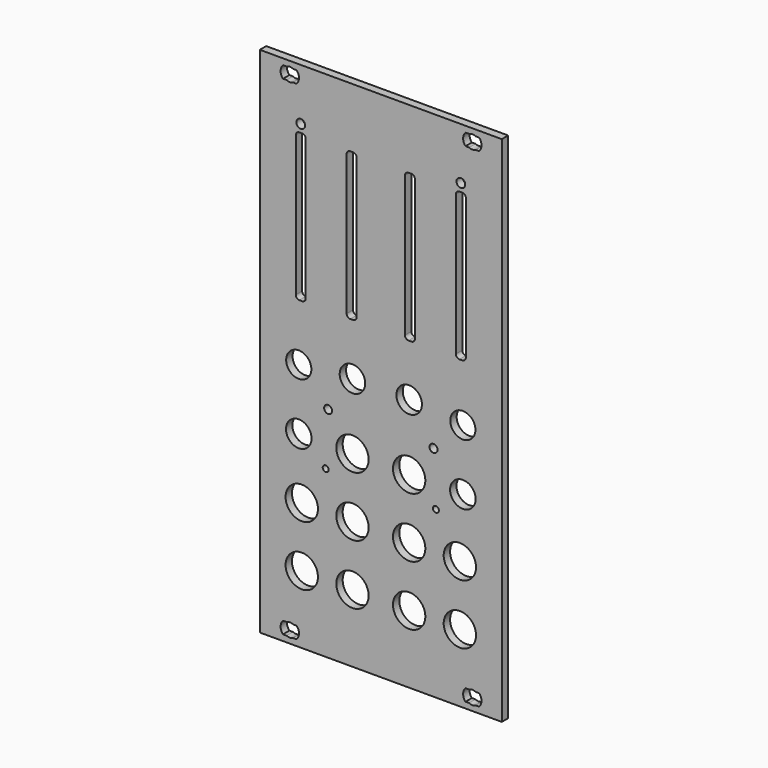
from build123d import *

# Parameters (mm, degrees)
F0_R     = 4.05
F0_R_2   = 3.200001
F0_R_3   = 3.15
F0_R_4   = 0.75
F0_R_5   = 1
F0_R_6   = 1.1
F1_DEPTH = 2


# Not quite as in the source:
# - ends of sketch curves that miss each other by under 0.0002 mm in the source are joined


with BuildPart() as f1:
    # F0 (on Front) → F1 (new body)
    with BuildSketch(Plane.XZ):
        Polygon((-30.3, -61.250013), (-30.3, -64.250012), (30.300001, -64.250012), (30.300001, 64.250011), (-30.3, 64.250011), align=None)
        with BuildLine():
            ThreePointArc((-23.600001, -59.750013), (-22.7999995588, -59.550011), (-21.9999982215, -59.7500134152))
            Line((-21.9999982215, -59.7500134152), (-21.100001, -59.750013))
            ThreePointArc((-21.100001, -59.750013), (-20.5, -61.2500126379), (-21.1000001998, -62.7500108097))
            Line((-21.1000001998, -62.7500108097), (-21.999999, -62.750012))
            ThreePointArc((-21.999999, -62.750012), (-22.7999995588, -62.950014), (-23.600001, -62.750012))
            Line((-23.600001, -62.750012), (-24.499999, -62.750012))
            ThreePointArc((-24.499999, -62.750012), (-25.1, -61.2500126379), (-24.4999988252, -59.7500141665))
            Line((-24.4999988252, -59.7500141665), (-23.600001, -59.750013))
        make_face(mode=Mode.SUBTRACT)
        with Locations((-19.800001, -47.249931)):
            Circle(F0_R, mode=Mode.SUBTRACT)
        with Locations((-19.800052, -32.249984)):
            Circle(F0_R, mode=Mode.SUBTRACT)
        with Locations((-7.100001, -47.249931)):
            Circle(F0_R, mode=Mode.SUBTRACT)
        with Locations((-7.100052, -32.249984)):
            Circle(F0_R, mode=Mode.SUBTRACT)
        with Locations((-20.549999, -17.249989)):
            Circle(F0_R_2, mode=Mode.SUBTRACT)
        with Locations((-20.549999, -1.999989)):
            Circle(F0_R_3, mode=Mode.SUBTRACT)
        with Locations((-13.8, -22.749991)):
            Circle(F0_R_4, mode=Mode.SUBTRACT)
        with Locations((-7.100052, -17.249986)):
            Circle(F0_R, mode=Mode.SUBTRACT)
        with Locations((-13.200001, -9.499989)):
            Circle(F0_R_5, mode=Mode.SUBTRACT)
        with Locations((-7.100001, -0.749989)):
            Circle(F0_R_2, mode=Mode.SUBTRACT)
        with Locations((7.099976, -47.249957)):
            Circle(F0_R, mode=Mode.SUBTRACT)
        with Locations((7.09995, -32.249928)):
            Circle(F0_R, mode=Mode.SUBTRACT)
        with BuildLine():
            ThreePointArc((22.119986, -59.750023), (22.9199874412, -59.550021), (23.7199887785, -59.7500234152))
            Line((23.7199887785, -59.7500234152), (24.619987, -59.750023))
            ThreePointArc((24.619987, -59.750023), (25.219987, -61.250023), (24.6199863008, -62.7500213341))
            Line((24.6199863008, -62.7500213341), (23.719988, -62.750022))
            ThreePointArc((23.719988, -62.750022), (22.9199874412, -62.950024), (22.119986, -62.750022))
            Line((22.119986, -62.750022), (21.219988, -62.750022))
            ThreePointArc((21.219988, -62.750022), (20.619987, -61.250023), (21.2199901249, -59.7500221189))
            Line((21.2199901249, -59.7500221189), (22.119986, -59.750023))
        make_face(mode=Mode.SUBTRACT)
        with Locations((19.799976, -47.249957)):
            Circle(F0_R, mode=Mode.SUBTRACT)
        with Locations((19.79995, -32.249928)):
            Circle(F0_R, mode=Mode.SUBTRACT)
        with Locations((7.099925, -17.249928)):
            Circle(F0_R, mode=Mode.SUBTRACT)
        with Locations((13.799975, -22.749991)):
            Circle(F0_R_4, mode=Mode.SUBTRACT)
        with Locations((7.100052, -0.749989)):
            Circle(F0_R_2, mode=Mode.SUBTRACT)
        with Locations((13.199999, -9.499989)):
            Circle(F0_R_5, mode=Mode.SUBTRACT)
        with Locations((20.549974, -17.249989)):
            Circle(F0_R_2, mode=Mode.SUBTRACT)
        with Locations((20.549974, -1.999989)):
            Circle(F0_R_3, mode=Mode.SUBTRACT)
        with BuildLine():
            Line((-21.3, 13.150011), (-21.3, 30.750012))
            Line((-21.3, 30.750012), (-21.3, 48.350012))
            ThreePointArc((-21.3, 48.350012), (-21.0363968102, 48.9864088102), (-20.4, 49.250013))
            Line((-20.4, 49.250013), (-19.700001, 49.250013))
            ThreePointArc((-19.700001, 49.250013), (-19.0636041898, 48.9864088102), (-18.8, 48.350012))
            Line((-18.8, 48.350012), (-18.8, 30.750012))
            Line((-18.8, 30.750012), (-18.8, 13.150011))
            ThreePointArc((-18.8, 13.150011), (-19.0636041898, 12.5136141898), (-19.700001, 12.25001))
            Line((-19.700001, 12.25001), (-20.4, 12.250011))
            ThreePointArc((-20.4, 12.250011), (-21.0363968102, 12.5136141898), (-21.3, 13.150011))
        make_face(mode=Mode.SUBTRACT)
        with BuildLine():
            Line((-8.55, 13.150011), (-8.55, 30.750012))
            Line((-8.55, 30.750012), (-8.55, 48.350012))
            ThreePointArc((-8.55, 48.350012), (-8.2863968102, 48.9864088102), (-7.65, 49.250013))
            Line((-7.65, 49.250013), (-6.950001, 49.250013))
            ThreePointArc((-6.950001, 49.250013), (-6.3136041898, 48.9864088102), (-6.05, 48.350012))
            Line((-6.05, 48.350012), (-6.05, 30.750012))
            Line((-6.05, 30.750012), (-6.05, 13.150011))
            ThreePointArc((-6.05, 13.150011), (-6.3136041898, 12.5136141898), (-6.950001, 12.25001))
            Line((-6.950001, 12.25001), (-7.65, 12.250011))
            ThreePointArc((-7.65, 12.250011), (-8.2863968102, 12.5136141898), (-8.55, 13.150011))
        make_face(mode=Mode.SUBTRACT)
        with BuildLine():
            ThreePointArc((-23.600014, 62.750001), (-22.8000125588, 62.950003), (-22.0000112215, 62.7500005848))
            Line((-22.0000112215, 62.7500005848), (-21.100013, 62.750001))
            ThreePointArc((-21.100013, 62.750001), (-20.500013, 61.2500013621), (-21.1000131998, 59.7500031903))
            Line((-21.1000131998, 59.7500031903), (-22.000012, 59.750002))
            ThreePointArc((-22.000012, 59.750002), (-22.8000125588, 59.55), (-23.600014, 59.750002))
            Line((-23.600014, 59.750002), (-24.500012, 59.750002))
            ThreePointArc((-24.500012, 59.750002), (-25.100013, 61.2500013621), (-24.5000093757, 62.7500024055))
            Line((-24.5000093757, 62.7500024055), (-23.600014, 62.750001))
        make_face(mode=Mode.SUBTRACT)
        with Locations((-20.049998, 51.250011)):
            Circle(F0_R_6, mode=Mode.SUBTRACT)
        with BuildLine():
            Line((6.050001, 13.150011), (6.050001, 30.750012))
            Line((6.050001, 30.750012), (6.050001, 48.350012))
            ThreePointArc((6.050001, 48.350012), (6.3136051898, 48.9864088102), (6.950002, 49.250013))
            Line((6.950002, 49.250013), (7.65, 49.250013))
            ThreePointArc((7.65, 49.250013), (8.2863968102, 48.9864088102), (8.550001, 48.350012))
            Line((8.550001, 48.350012), (8.550001, 30.750012))
            Line((8.550001, 30.750012), (8.550001, 13.150011))
            ThreePointArc((8.550001, 13.150011), (8.2863968102, 12.5136141898), (7.65, 12.25001))
            Line((7.65, 12.25001), (6.950002, 12.250011))
            ThreePointArc((6.950002, 12.250011), (6.3136051898, 12.5136141898), (6.050001, 13.150011))
        make_face(mode=Mode.SUBTRACT)
        with BuildLine():
            Line((18.800001, 13.150009), (18.800001, 30.750009))
            Line((18.800001, 30.750009), (18.800001, 48.35001))
            ThreePointArc((18.800001, 48.35001), (19.0636041898, 48.9864068102), (19.700001, 49.250011))
            Line((19.700001, 49.250011), (20.4, 49.25001))
            ThreePointArc((20.4, 49.25001), (21.0363968102, 48.9864068102), (21.300001, 48.35001))
            Line((21.300001, 48.35001), (21.300001, 30.750009))
            Line((21.300001, 30.750009), (21.300001, 13.150009))
            ThreePointArc((21.300001, 13.150009), (21.0363968102, 12.5136121898), (20.4, 12.250008))
            Line((20.4, 12.250008), (19.700001, 12.250008))
            ThreePointArc((19.700001, 12.250008), (19.0636041898, 12.5136121898), (18.800001, 13.150009))
        make_face(mode=Mode.SUBTRACT)
        with Locations((20.050001, 51.250009)):
            Circle(F0_R_6, mode=Mode.SUBTRACT)
        with BuildLine():
            Line((22.119986, 59.750002), (21.219988, 59.750002))
            ThreePointArc((21.219988, 59.750002), (20.619987, 61.2500013621), (21.2199906243, 62.7500024055))
            Line((21.2199906243, 62.7500024055), (22.119986, 62.750001))
            ThreePointArc((22.119986, 62.750001), (22.9199874412, 62.950003), (23.7199887785, 62.7500005848))
            Line((23.7199887785, 62.7500005848), (24.619987, 62.750001))
            ThreePointArc((24.619987, 62.750001), (25.219987, 61.2500013621), (24.6199868002, 59.7500031903))
            Line((24.6199868002, 59.7500031903), (23.719988, 59.750002))
            ThreePointArc((23.719988, 59.750002), (22.9199874412, 59.55), (22.119986, 59.750002))
        make_face(mode=Mode.SUBTRACT)
    extrude(amount=F1_DEPTH)


solid = f1.part
